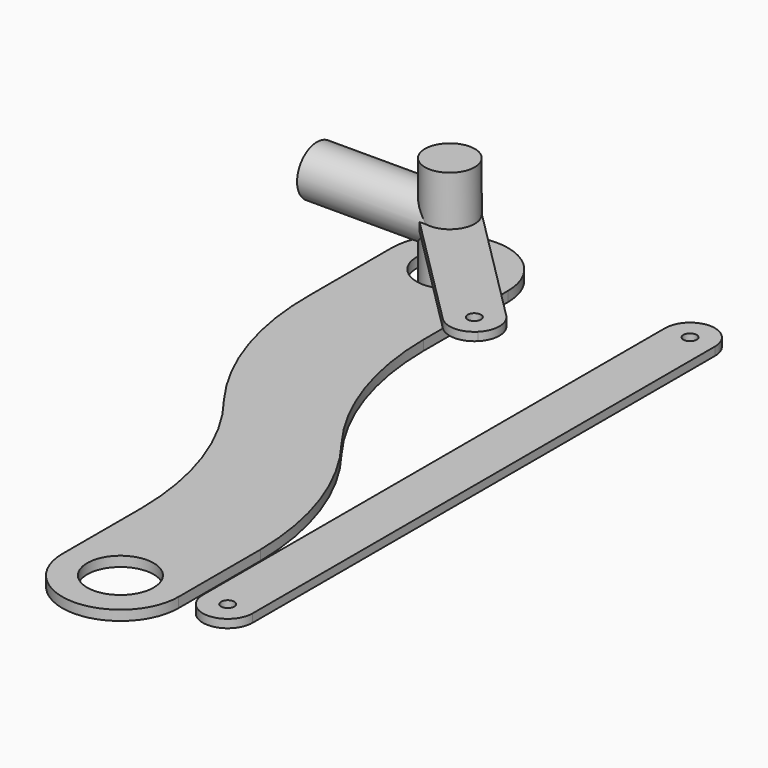
from build123d import *

# Parameters (mm, degrees)
F0_R      = 20
F1_DEPTH  = 6
F2_R      = 15
F3_DEPTH  = 65
F4_R      = 15
F5_DEPTH  = 80
F7_W      = 30
F7_H      = 5
F8_DEPTH  = 120
F10_D     = 8
F11_R     = 14.99999
F13_DEPTH = 5
F14_D     = 8


# Not quite as in the source:
# - a fillet or chamfer is up to 0.001 mm smaller than in the source, because OpenCascade refuses the exact size


with BuildPart() as f1:
    # F0 (on Top) → F1 (new body)
    with BuildSketch(Plane.XY):
        with BuildLine():
            Line((-35, 0), (-35, -61.0286490145))
            ThreePointArc((-35, -61.0286490145), (-26.3919474837, -118.3702876491), (0, -170))
            ThreePointArc((0, -170), (28.5488738406, -221.9245845611), (38.6905676698, -280.3056322195))
            ThreePointArc((38.6905676698, -280.3056322195), (38.6945456991, -281.5023254682), (38.6905676698, -282.6990187168))
            Line((38.6905676698, -282.6990187168), (38.6905676698, -340))
            ThreePointArc((38.6905676698, -340), (73.6905676698, -375), (108.6905676698, -340))
            Line((108.6905676698, -340), (108.6905676698, -282.6990187168))
            Line((108.6905676698, -282.6990187168), (108.6905676698, -278.31146671))
            ThreePointArc((108.6905676698, -278.31146671), (98.6028154032, -221.0546666233), (70.7904994631, -170))
            ThreePointArc((70.7904994631, -170), (44.3760227078, -119.6233145812), (35, -63.5196140416))
            Line((35, -63.5196140416), (35, 0))
            ThreePointArc((35, 0), (0, 35), (-35, 0))
        make_face()
        with Locations((73.6905676698, -340)):
            Circle(F0_R, mode=Mode.SUBTRACT)
        Circle(F0_R, mode=Mode.SUBTRACT)
    extrude(amount=F1_DEPTH)


with BuildPart() as f3:
    # F2 (on Top) → F3 (new body)
    with BuildSketch(Plane.XY):
        Circle(F2_R)
    extrude(amount=F3_DEPTH)

    # F4 (on Right) → F5 (join)
    with BuildSketch(Plane.YZ):
        with Locations((0, 32.5)):
            Circle(F4_R)
    extrude(amount=-F5_DEPTH)

    # F7 (on face) → F8 (join)
    with BuildSketch(Plane(origin=(0, 0, 0), x_dir=(0.7071067812, 0.7071067812, 0), z_dir=(0.7071067812, -0.7071067812, 0))):
        with Locations((0, 32.5)):
            Rectangle(F7_W, F7_H)
    extrude(amount=F8_DEPTH)

    # F10 (through all)
    with Locations(Plane(origin=(0, 0, 0), x_dir=(1, 0, 0), z_dir=(0, 0, -1))):
        with Locations((74.1714673688, 74.321487157)):
            Hole(F10_D / 2)

    # F11 (radius 15 in the source; OpenCascade refuses exactly that, so slightly less here)
    f11_edges = [f3.edges().sort_by_distance(p)[0] for p in [
        (95.459415, -74.246212, 32.5),
        (74.246212, -95.459415, 32.5),
    ]]
    fillet(f11_edges, radius=F11_R)


with BuildPart() as f13:
    # F12 (on Top) → F13 (new body)
    with BuildSketch(Plane.XY):
        with BuildLine():
            ThreePointArc((130.1932446659, 32.9991710233), (119.5866429481, 28.6057727411), (115.1932446659, 17.9991710233))
            Line((115.1932446659, 17.9991710233), (115.1932446659, -329.8949189767))
            ThreePointArc((115.1932446659, -329.8949189767), (119.5866429481, -340.5015206945), (130.1932446659, -344.8949189767))
            ThreePointArc((130.1932446659, -344.8949189767), (140.7998463837, -340.5015206945), (145.1932446659, -329.8949189767))
            Line((145.1932446659, -329.8949189767), (145.1932446659, 17.9991710233))
            ThreePointArc((145.1932446659, 17.9991710233), (140.7998463837, 28.6057727411), (130.1932446659, 32.9991710233))
        make_face()
    extrude(amount=F13_DEPTH)

    # F14 (through all)
    with Locations(Plane(origin=(0, 0, 0), x_dir=(1, 0, 0), z_dir=(0, 0, -1))):
        with Locations((130.1932446659, 329.8949189767), (130.1932446659, -17.9991710233)):
            Hole(F14_D / 2)


solid = Compound([f1.part, f3.part, f13.part])
